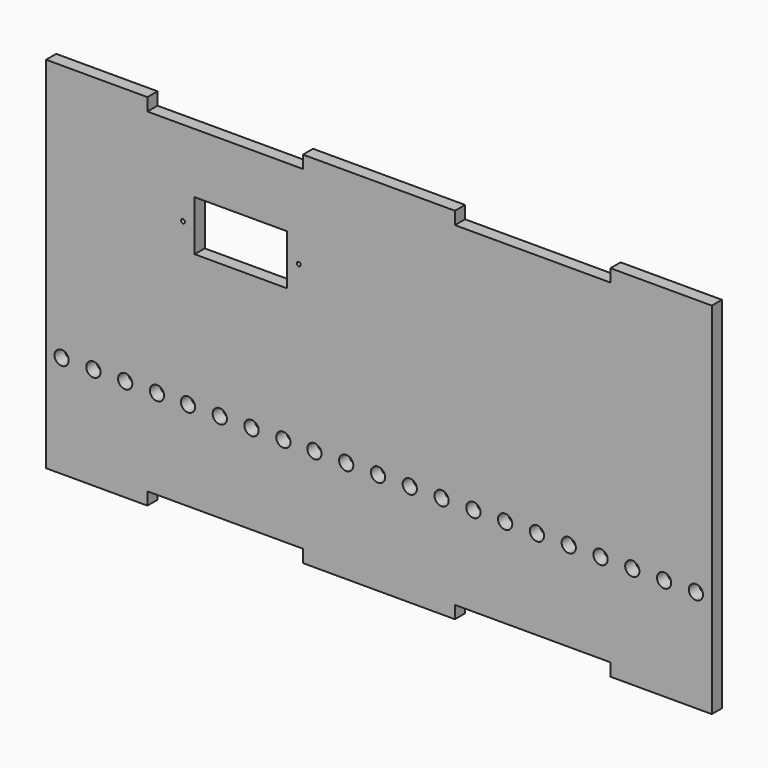
from build123d import *

# Parameters (mm, degrees)
F0_R     = 1.7859375
F0_R_2   = 0.5
F0_W     = 23.2
F0_H     = 12.6
F1_DEPTH = 3.175


# Not quite as in the source:
# - a length typed as a fraction of an inch, garbled in the dataset ("3 / 203.2 mm" for 3/8 in), is restored


with BuildPart() as f1:
    # F0 (on Front) → F1 (new body)
    with BuildSketch(Plane.XZ):
        Polygon((-67.2774, 61.1329712169), (-67.2774, -22.4699976), (-67.2774, -25.6449976), (-41.8774, -25.6449976), (-41.8774, -22.4699976), (-2.8762, -22.4699976), (-2.8762, -25.6449976), (35.2238, -25.6449976), (35.2238, -22.4699976), (74.225, -22.4699976), (74.225, -25.6449976), (99.625, -25.6449976), (99.625, -22.4699976), (99.625, 61.3500024), (99.625, 64.5250024), (74.225, 64.5250024), (74.225, 61.3500024), (35.2238, 61.3500024), (35.2238, 64.5250024), (-2.8762, 64.5250024), (-2.8762, 61.3500024), (-41.8774, 61.3500024), (-41.8774, 64.5250024), (-67.2774, 64.5250024), (-67.2774, 61.3500024), align=None)
        with Locations((-63.3824, 0)):
            Circle(F0_R, mode=Mode.SUBTRACT)
        with Locations((-55.4124, 0)):
            Circle(F0_R, mode=Mode.SUBTRACT)
        with Locations((-47.4424, 0)):
            Circle(F0_R, mode=Mode.SUBTRACT)
        with Locations((-39.4724, 0)):
            Circle(F0_R, mode=Mode.SUBTRACT)
        with Locations((-31.7, 0)):
            Circle(F0_R, mode=Mode.SUBTRACT)
        with Locations((-23.73, 0)):
            Circle(F0_R, mode=Mode.SUBTRACT)
        with Locations((-15.76, 0)):
            Circle(F0_R, mode=Mode.SUBTRACT)
        with Locations((-7.79, 0)):
            Circle(F0_R, mode=Mode.SUBTRACT)
        Circle(F0_R, mode=Mode.SUBTRACT)
        with Locations((7.97, 0)):
            Circle(F0_R, mode=Mode.SUBTRACT)
        with Locations((15.94, 0)):
            Circle(F0_R, mode=Mode.SUBTRACT)
        with Locations((23.91, 0)):
            Circle(F0_R, mode=Mode.SUBTRACT)
        with Locations((31.88, 0)):
            Circle(F0_R, mode=Mode.SUBTRACT)
        with Locations((39.85, 0)):
            Circle(F0_R, mode=Mode.SUBTRACT)
        with Locations((47.82, 0)):
            Circle(F0_R, mode=Mode.SUBTRACT)
        with Locations((55.79, 0)):
            Circle(F0_R, mode=Mode.SUBTRACT)
        with Locations((63.76, 0)):
            Circle(F0_R, mode=Mode.SUBTRACT)
        with Locations((71.73, 0)):
            Circle(F0_R, mode=Mode.SUBTRACT)
        with Locations((79.7, 0)):
            Circle(F0_R, mode=Mode.SUBTRACT)
        with Locations((87.67, 0)):
            Circle(F0_R, mode=Mode.SUBTRACT)
        with Locations((95.64, 0)):
            Circle(F0_R, mode=Mode.SUBTRACT)
        with Locations((-32.93, 40.005)):
            Circle(F0_R_2, mode=Mode.SUBTRACT)
        with Locations((-18.43, 40.005)):
            Rectangle(F0_W, F0_H, mode=Mode.SUBTRACT)
        with Locations((-3.93, 40.005)):
            Circle(F0_R_2, mode=Mode.SUBTRACT)
    extrude(amount=F1_DEPTH)


solid = f1.part
